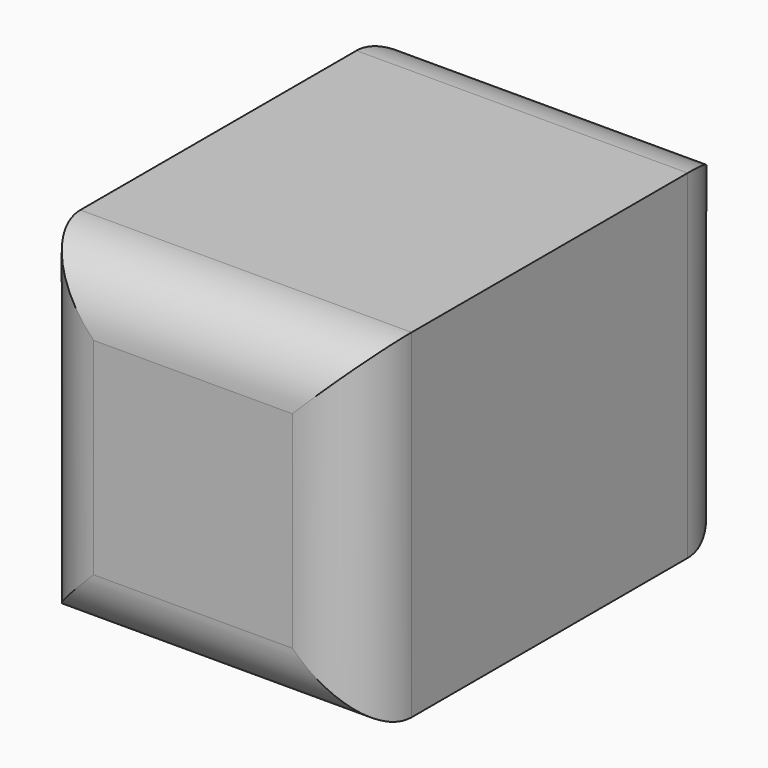
from build123d import *

# Parameters (mm, degrees)
F0_W        = 36.6208925843
F0_H        = 25.9851198643
F1_DEPTH    = 25.4
F3_DEPTH    = 12.7
F4_DEPTH    = 12.7
F5_T1_DEPTH = 50.8
F5_T3_DEPTH = 51.3851198643
F6_T1_DEPTH = 50.8
F6_T3_DEPTH = 51.3851198643


# Not quite as in the source:
# - a fillet or chamfer that OpenCascade refuses, or shapes differently, is made with other operations: its cross-section is extruded or revolved along the edge and cut away or added


with BuildPart() as f1:
    # F0 (on Right) → F1 (new body)
    with BuildSketch(Plane.YZ):
        with Locations((-18.3104462922, 12.9925599322)):
            Rectangle(F0_W, F0_H)
    extrude(amount=F1_DEPTH)

    # F2 (on Top) → F3 (join)
    with BuildSketch(Plane.XY):
        Polygon((20.2587246895, -3.5579784308), (4.1429102421, -3.3661234193), (4.1429102421, -32.3362164199), (20.2587246895, -32.3362164199), align=None)
    extrude(amount=F3_DEPTH)

    # F2 (on Top) → F4 (cut)
    with BuildSketch(Plane.XY):
        Polygon((20.2587246895, -3.5579784308), (4.1429102421, -3.3661234193), (4.1429102421, -32.3362164199), (20.2587246895, -32.3362164199), align=None)
    extrude(amount=F4_DEPTH, mode=Mode.SUBTRACT)

    # F5: fillet of radius 5.08 on 4 edges, made by hand

    # F5_s2 → F5_t1 (cut)
    with BuildSketch(Plane.YZ.offset(-12.7)):
        with BuildLine():
            ThreePointArc((-36.6208925843, 20.9051198643), (-35.1329950328, 24.4972223128), (-31.5408925843, 25.9851198643))
            Line((-31.5408925843, 25.9851198643), (-36.6208925843, 25.9851198643))
            Line((-36.6208925843, 25.9851198643), (-36.6208925843, 20.9051198643))
        make_face()
        with BuildLine():
            ThreePointArc((-31.5408925843, 0), (-35.1329950328, 1.4878975516), (-36.6208925843, 5.08))
            Line((-36.6208925843, 5.08), (-36.6208925843, 0))
            Line((-36.6208925843, 0), (-31.5408925843, 0))
        make_face()
    extrude(amount=F5_T1_DEPTH, mode=Mode.SUBTRACT)

    # F5_s4 → F5_t3 (cut)
    with BuildSketch(Plane.XY.offset(-12.7)):
        with BuildLine():
            ThreePointArc((5.08, -36.6208925843), (1.4878975516, -35.1329950328), (0, -31.5408925843))
            Line((0, -31.5408925843), (0, -36.6208925843))
            Line((0, -36.6208925843), (5.08, -36.6208925843))
        make_face()
        with BuildLine():
            ThreePointArc((20.32, -36.6208925843), (23.9121024484, -35.1329950328), (25.4, -31.5408925843))
            Line((25.4, -31.5408925843), (25.4, -36.6208925843))
            Line((25.4, -36.6208925843), (20.32, -36.6208925843))
        make_face()
    extrude(amount=F5_T3_DEPTH, mode=Mode.SUBTRACT)

    # F6: fillet of radius 5.08 on 4 edges, made by hand

    # F6_s2 → F6_t1 (cut)
    with BuildSketch(Plane.YZ.offset(-12.7)):
        with BuildLine():
            ThreePointArc((-5.08, 0), (-1.4878975516, 1.4878975516), (0, 5.08))
            Line((0, 5.08), (0, 0))
            Line((0, 0), (-5.08, 0))
        make_face()
        with BuildLine():
            ThreePointArc((0, 20.9051198643), (-1.4878975516, 24.4972223128), (-5.08, 25.9851198643))
            Line((-5.08, 25.9851198643), (0, 25.9851198643))
            Line((0, 25.9851198643), (0, 20.9051198643))
        make_face()
    extrude(amount=F6_T1_DEPTH, mode=Mode.SUBTRACT)

    # F6_s4 → F6_t3 (cut)
    with BuildSketch(Plane.XY.offset(-12.7)):
        with BuildLine():
            ThreePointArc((0, -5.08), (1.4878975516, -1.4878975516), (5.08, 0))
            Line((5.08, 0), (0, 0))
            Line((0, 0), (0, -5.08))
        make_face()
        with BuildLine():
            ThreePointArc((20.32, 0), (23.9121024484, -1.4878975516), (25.4, -5.08))
            Line((25.4, -5.08), (25.4, 0))
            Line((25.4, 0), (20.32, 0))
        make_face()
    extrude(amount=F6_T3_DEPTH, mode=Mode.SUBTRACT)


solid = f1.part
